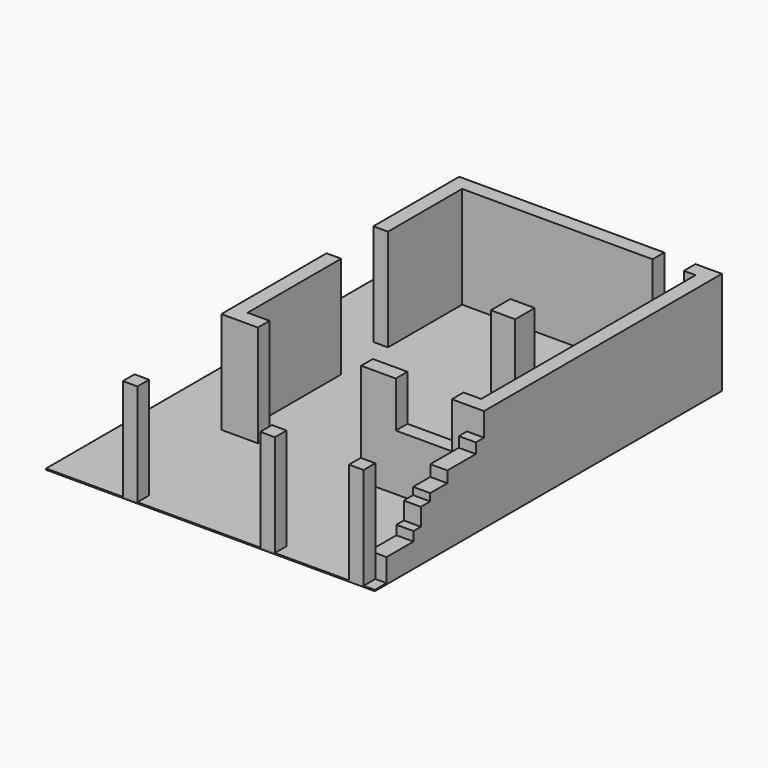
from build123d import *

# Parameters (mm, degrees)
F0_W      = 350
F0_H      = 210
F1_DEPTH  = 1610
F0_H_2    = 730
F2_DEPTH  = 1400
F0_H_3    = 440
F3_DEPTH  = 1170
F0_H_4    = 240
F4_DEPTH  = 1020
F0_H_5    = 190
F5_DEPTH  = 660
F6_DEPTH  = 470
F0_W_2    = 300
F0_H_6    = 300
F7_DEPTH  = 2090
F8_DEPTH  = 2090
F0_W_3    = 500
F0_H_7    = 500
F0_W_4    = 710
F10_DEPTH = 25
F11_W     = 1150
F11_H     = 300
F12_DEPTH = 1150


# Not quite as in the source:
# - a feature of the source that left no trace in its solid (it failed there, or was rolled back) is left out


with BuildPart() as f1:
    # F0 (on Top) → F1 (new body)
    with BuildSketch(Plane.XY):
        with Locations((2365.7681007385, -3318.20271492)):
            Rectangle(F0_W, F0_H)
    extrude(amount=F1_DEPTH)

    # F0 (on Top) → F2 (join)
    with BuildSketch(Plane.XY):
        with Locations((2365.7681007385, -3788.20271492)):
            Rectangle(F0_W, F0_H_2)
    extrude(amount=F2_DEPTH)

    # F0 (on Top) → F3 (join)
    with BuildSketch(Plane.XY):
        with Locations((2365.7681007385, -4373.20271492)):
            Rectangle(F0_W, F0_H_3)
    extrude(amount=F3_DEPTH)

    # F0 (on Top) → F4 (join)
    with BuildSketch(Plane.XY):
        with Locations((2365.7681007385, -4713.20271492)):
            Rectangle(F0_W, F0_H_4)
    extrude(amount=F4_DEPTH)

    # F0 (on Top) → F5 (join)
    with BuildSketch(Plane.XY):
        with Locations((2365.7681007385, -4928.20271492)):
            Rectangle(F0_W, F0_H_5)
    extrude(amount=F5_DEPTH)

    # F0 (on Top) → F6 (join)
    with BuildSketch(Plane.XY):
        Polygon((2540.7681007385, -5023.20271492), (2190.7681007385, -5023.20271492), (2190.7681007385, -5713.20271492), (2310.7681007385, -5713.20271492), (2540.7681007385, -5713.20271492), align=None)
    extrude(amount=F6_DEPTH)

    # F0 (on Top) → F7, piece 3 (join)
    with BuildSketch(Plane.XY):
        Polygon((2310.7681007385, -5713.20271492), (2190.7681007385, -5713.20271492), (2010.7681007385, -5713.20271492), (2010.7681007385, -6013.20271492), (2310.7681007385, -6013.20271492), align=None)
    extrude(amount=F7_DEPTH)

    # F0 (on Top) → F8, piece 5 (join)
    with BuildSketch(Plane.XY):
        Polygon((2240.7681007385, -2913.20271492), (1880.7681007385, -2913.20271492), (1880.7681007385, -3213.20271492), (2190.7681007385, -3213.20271492), (2540.7681007385, -3213.20271492), (2540.7681007385, 2886.79728508), (1999.1303939819, 2886.79728508), (1999.1303939819, 2586.79728508), (2240.7681007385, 2586.79728508), align=None)
    extrude(amount=F8_DEPTH)



with BuildPart() as f7:
    # F0 (on Top) → F7 (new body)
    with BuildSketch(Plane.XY):
        with Locations((-2479.2318992615, -5863.20271492)):
            Rectangle(F0_W_2, F0_H_6)
    extrude(amount=F7_DEPTH)


with BuildPart() as f7b:
    # F0 (on Top) → F7, piece 2 (new body)
    with BuildSketch(Plane.XY):
        with Locations((340.7681007385, -5863.20271492)):
            Rectangle(F0_W_2, F0_H_6)
    extrude(amount=F7_DEPTH)


with BuildPart() as f8:
    # F0 (on Top) → F8 (new body)
    with BuildSketch(Plane.XY):
        Polygon((-2849.2318992615, 686.79728508), (-2549.2318992615, 686.79728508), (-2549.2318992615, 2586.79728508), (1357.8613657951, 2586.79728508), (1357.8613657951, 2886.79728508), (-2849.2318992615, 2886.79728508), align=None)
    extrude(amount=F8_DEPTH)


with BuildPart() as f8b:
    # F0 (on Top) → F8, piece 2 (new body)
    with BuildSketch(Plane.XY):
        with Locations((690.7681007385, -163.20271492)):
            Rectangle(F0_W_3, F0_H_7)
    extrude(amount=F8_DEPTH)


with BuildPart() as f8c:
    # F0 (on Top) → F8, piece 3 (new body)
    with BuildSketch(Plane.XY):
        Polygon((-2099.2318992615, -2913.20271492), (-2549.2318992615, -2913.20271492), (-2549.2318992615, -513.20271492), (-2849.2318992615, -513.20271492), (-2849.2318992615, -3213.20271492), (-2099.2318992615, -3213.20271492), align=None)
    extrude(amount=F8_DEPTH)


with BuildPart() as f8d:
    # F0 (on Top) → F8, piece 4 (new body)
    with BuildSketch(Plane.XY):
        with Locations((375.7681007385, -3063.20271492)):
            Rectangle(F0_W_4, F0_H_6)
    extrude(amount=F8_DEPTH)


with BuildPart() as f1_1:
    add(f1.part)

    add(f8d.part)  # F10 merges F8d
    # F9 (on face) → F10 (join)
    with BuildSketch(Plane(origin=(0, 0, 0), x_dir=(1, 0, 0), z_dir=(0, 0, -1))):
        Polygon((-4202.8398513794, -2886.79728508), (-2849.2318992615, -2886.79728508), (-2849.2318992615, -686.79728508), (-2549.2318992615, -686.79728508), (-2549.2318992615, -2586.79728508), (1357.8613657951, -2586.79728508), (1357.8613657951, -2886.79728508), (2540.7681007385, -2886.79728508), (2540.7681007385, 6013.20271492), (-2849.2318992615, 6013.20271492), (-4202.8398513794, 6013.20271492), align=None)
        Polygon((-2849.2318992615, -686.79728508), (-2849.2318992615, -2886.79728508), (1357.8613657951, -2886.79728508), (1357.8613657951, -2586.79728508), (-2549.2318992615, -2586.79728508), (-2549.2318992615, -686.79728508), align=None)
    extrude(amount=F10_DEPTH)

    # F11 (on face) → F12 (join)
    with BuildSketch(Plane.XY):
        with Locations((1305.7681007385, -3063.20271492)):
            Rectangle(F11_W, F11_H)
    extrude(amount=F12_DEPTH)


solid = Compound([f7.part, f7b.part, f8.part, f8b.part, f8c.part, f1_1.part])
